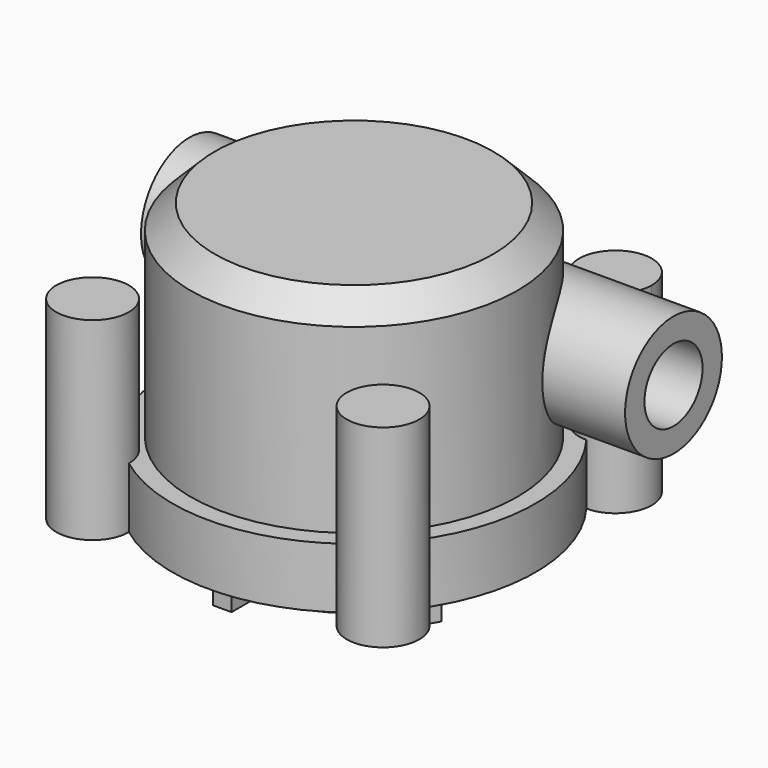
from build123d import *

# Parameters (mm, degrees)
F0_R      = 15
F1_DEPTH  = 5
F2_R      = 3
F3_DEPTH  = 16
F6_R      = 13.5
F7_DEPTH  = 17
F8_SIZE   = 2
F5_R      = 5
F5_R_2    = 3
F9_DEPTH  = 20
F11_DEPTH = 2


with BuildPart() as f1:
    # F0 (on Top) → F1 (new body)
    with BuildSketch(Plane.XY):
        Circle(F0_R)
    extrude(amount=F1_DEPTH)

    # F2 (on face) → F3 (join)
    with BuildSketch(Plane(origin=(0, 0, 0), x_dir=(1, 0, 0), z_dir=(0, 0, -1))):
        with Locations((12, -12)):
            Circle(F2_R)
        with Locations((-12, -12)):
            Circle(F2_R)
        with Locations((-12, 12)):
            Circle(F2_R)
        with Locations((12, 12)):
            Circle(F2_R)
    extrude(amount=-F3_DEPTH)

    # F6 (on face) → F7 (join)
    with BuildSketch(Plane.XY.offset(5)):
        Circle(F6_R)
    extrude(amount=F7_DEPTH)

    # F8
    f8_edges = [f1.edges().sort_by_distance(p)[0] for p in [
        (-13.5, 0, 22),
    ]]
    chamfer(f8_edges, length=F8_SIZE)

    # F5 (on Right) → F9 (join, symmetric)
    with BuildSketch(Plane.YZ):
        with Locations((8, 12)):
            Circle(F5_R)
        with Locations((8, 12)):
            Circle(F5_R_2, mode=Mode.SUBTRACT)
    extrude(amount=F9_DEPTH, both=True)

    # F10 (on face) → F11 (join)
    with BuildSketch(Plane(origin=(0, 0, 0), x_dir=(1, 0, 0), z_dir=(0, 0, -1))):
        with BuildLine():
            Line((0.7608169108, -13.6017159084), (0.7608169108, -11.2095828595))
            ThreePointArc((0.7608169108, -11.2095828595), (5.6176861397, -9.7301178149), (9.3273750667, -6.2636782021))
            Line((9.3273750667, -6.2636782021), (11.3990230563, -7.4597447266))
            Line((11.3990230563, -7.4597447266), (12.1598399671, -6.1419711818))
            Line((12.1598399671, -6.1419711818), (10.0881919775, -4.9459046574))
            ThreePointArc((10.0881919775, -4.9459046574), (11.2353722793, 0), (10.0881919775, 4.9459046574))
            Line((10.0881919775, 4.9459046574), (12.1598399671, 6.1419711818))
            Line((12.1598399671, 6.1419711818), (11.3990230563, 7.4597447266))
            Line((11.3990230563, 7.4597447266), (9.3273750667, 6.2636782021))
            ThreePointArc((9.3273750667, 6.2636782021), (5.6176861397, 9.7301178149), (0.7608169108, 11.2095828595))
            Line((0.7608169108, 11.2095828595), (0.7608169108, 13.6017159084))
            Line((0.7608169108, 13.6017159084), (-0.7608169108, 13.6017159084))
            Line((-0.7608169108, 13.6017159084), (-0.7608169108, 11.2095828595))
            ThreePointArc((-0.7608169108, 11.2095828595), (-5.6176861397, 9.7301178149), (-9.3273750667, 6.2636782021))
            Line((-9.3273750667, 6.2636782021), (-11.3990230563, 7.4597447266))
            Line((-11.3990230563, 7.4597447266), (-12.1598399671, 6.1419711818))
            Line((-12.1598399671, 6.1419711818), (-10.0881919775, 4.9459046574))
            ThreePointArc((-10.0881919775, 4.9459046574), (-11.2353722793, 0), (-10.0881919775, -4.9459046574))
            Line((-10.0881919775, -4.9459046574), (-12.1598399671, -6.1419711818))
            Line((-12.1598399671, -6.1419711818), (-11.3990230563, -7.4597447266))
            Line((-11.3990230563, -7.4597447266), (-9.3273750667, -6.2636782021))
            ThreePointArc((-9.3273750667, -6.2636782021), (-5.6176861397, -9.7301178149), (-0.7608169108, -11.2095828595))
            Line((-0.7608169108, -11.2095828595), (-0.7608169108, -13.6017159084))
            Line((-0.7608169108, -13.6017159084), (0.7608169108, -13.6017159084))
        make_face()
    extrude(amount=F11_DEPTH)


solid = f1.part
